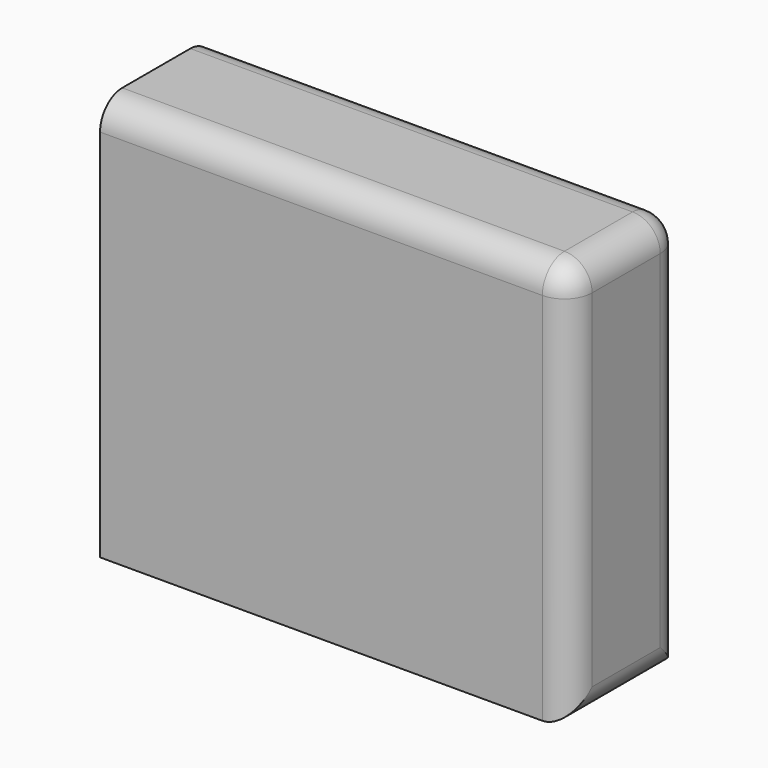
from build123d import *

# Parameters (mm, degrees)
F0_W     = 85.001712665
F0_H     = 72.736363858
F1_DEPTH = 25.4
F2_R     = 5
F3_R     = 5


with BuildPart() as f1:
    # F0 (on Front) → F1 (new body)
    with BuildSketch(Plane.XZ):
        with Locations((-16.5439592674, 2.8524082154)):
            Rectangle(F0_W, F0_H)
    extrude(amount=F1_DEPTH)

    # F2
    f2_edges = [f1.edges().sort_by_distance(p)[0] for p in [
        (25.956897, -12.7, 39.22059),
    ]]
    fillet(f2_edges, radius=F2_R)

    # F3
    f3_edges = [f1.edges().sort_by_distance(p)[0] for p in [
        (25.956897, 0, 0.352408),
        (25.956897, -12.7, 34.22059),
        (25.956897, -12.7, -33.515774),
        (25.956897, -25.4, 0.352408),
        (20.956897, -12.7, 39.22059),
    ]]
    fillet(f3_edges, radius=F3_R)


solid = f1.part
